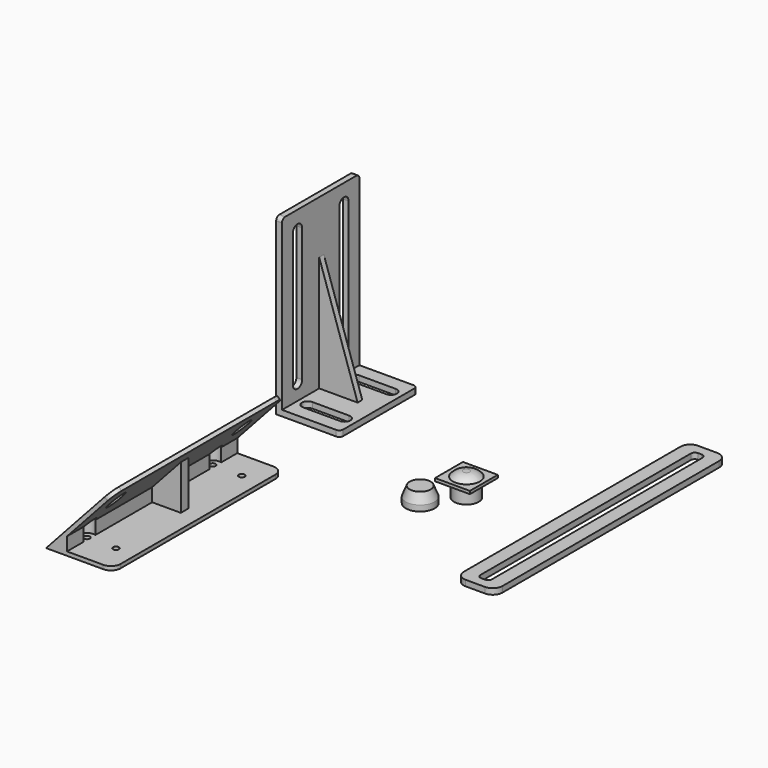
from build123d import *

# Parameters (mm, degrees)
F0_R        = 7
F1_DEPTH    = 2.5
F4_W        = 18
F4_H        = 18
F5_DEPTH    = 1.5
F7_R        = 6.4
F8_DEPTH    = 8
F9_R        = 7.45
F10_DEPTH   = 8
F11_SIZE2   = 5
F11_SIZE    = 2
F12_R       = 6.45
F13_DEPTH   = 7
F14_SIZE2   = 4
F14_SIZE    = 1.7
F17_DEPTH   = 3
F19_DEPTH   = 3
F20_W       = 3
F20_H       = 50
F21_DEPTH   = 90
F22_R       = 2
F24_DEPTH   = 25
F26_DEPTH   = 25
F29_DEPTH   = 3
F31_DEPTH   = 2
F33_DEPTH   = 110
F34_R       = 5
F36_DEPTH   = 110
F39_D       = 3
F39_DEPTH   = 50
F39_START   = 24.7920605
F39_START_2 = 41.2055101
F39_TIP     = 0.9012909285
F41_D       = 8
F41_DEPTH   = 19
F41_START   = 27.5276354
F41_START_2 = 43.9410851
F41_TIP     = 2.4034424761
F42_R       = 4
F43_DEPTH   = 2
F45_D       = 3
F45_DEPTH   = 19
F45_TIP     = 0.9012909285
F48_DEPTH   = 5


# Not quite as in the source:
# - a fillet or chamfer that OpenCascade refuses, or shapes differently, is made with other operations: its cross-section is extruded or revolved along the edge and cut away or added


with BuildPart() as f1:
    # F0 (on Top) → F1 (new body)
    with BuildSketch(Plane.XY):
        Circle(F0_R)
    extrude(amount=F1_DEPTH)

    # F2: fillet of radius 7 on 1 edges, made by hand

    # F2_s1 → F2_t2 (revolve, cut)
    with BuildSketch(Plane.XZ):
        with BuildLine():
            ThreePointArc((7, 0), (4.5961372442, 1.8442887702), (1.6380973526, 2.5))
            Line((1.6380973526, 2.5), (7, 2.5))
            Line((7, 2.5), (7, 0))
        make_face()
    revolve(axis=Axis((0, 0, 2.5), (0, 0, 1)), mode=Mode.SUBTRACT)

    # F4 (on offset) → F5 (join)
    with BuildSketch(Plane(origin=(0, 0, 0), x_dir=(1, 0, 0), z_dir=(0, 0, -1))):
        Rectangle(F4_W, F4_H)
    extrude(amount=F5_DEPTH)

    # F7 (on offset) → F8 (join)
    with BuildSketch(Plane(origin=(0, 0, -1.5), x_dir=(1, 0, 0), z_dir=(0, 0, -1))):
        Circle(F7_R)
    extrude(amount=F8_DEPTH)


with BuildPart() as f10:
    # F9 (on Top) → F10 (new body)
    with BuildSketch(Plane.XY):
        with Locations((0, -29.8365864904)):
            Circle(F9_R)
    extrude(amount=F10_DEPTH)

    # F11
    f11_edges = [f10.edges().sort_by_distance(p)[0] for p in [
        (-7.45, -29.836586, 8),
    ]]
    f11_side = f10.faces().sort_by_distance((0, -29.836586, 8))[0]
    chamfer(f11_edges, length=F11_SIZE, length2=F11_SIZE2, reference=f11_side)


with BuildPart() as f13:
    # F12 (on Top) → F13 (new body)
    with BuildSketch(Plane.XY):
        with Locations((0, -29.8365864904)):
            Circle(F12_R)
    extrude(amount=F13_DEPTH)

    # F14
    f14_edges = [f13.edges().sort_by_distance(p)[0] for p in [
        (-6.45, -29.836586, 7),
    ]]
    f14_side = f13.faces().sort_by_distance((0, -29.836586, 7))[0]
    chamfer(f14_edges, length=F14_SIZE, length2=F14_SIZE2, reference=f14_side)


with BuildPart() as f10_1:
    add(f10.part)

    # F15: cut F13
    add(f13.part, mode=Mode.SUBTRACT)


with BuildPart() as f17:
    # F16 (on Top) → F17 (new body)
    with BuildSketch(Plane.XY):
        with BuildLine():
            Line((69.802095294, 74.7819127334), (59.802095294, 74.7819127334))
            ThreePointArc((59.802095294, 74.7819127334), (56.2665613881, 73.3174466393), (54.802095294, 69.7819127334))
            Line((54.802095294, 69.7819127334), (54.802095294, -70.2180872666))
            ThreePointArc((54.802095294, -70.2180872666), (56.2665613881, -73.7536211725), (59.802095294, -75.2180872666))
            Line((59.802095294, -75.2180872666), (69.802095294, -75.2180872666))
            ThreePointArc((69.802095294, -75.2180872666), (73.3376291999, -73.7536211725), (74.802095294, -70.2180872666))
            Line((74.802095294, -70.2180872666), (74.802095294, 69.7819127334))
            ThreePointArc((74.802095294, 69.7819127334), (73.3376291999, 73.3174466393), (69.802095294, 74.7819127334))
        make_face()
        with BuildLine():
            ThreePointArc((61.802095294, 67.7819127334), (62.3878817316, 69.1961262958), (63.802095294, 69.7819127334))
            Line((63.802095294, 69.7819127334), (65.802095294, 69.7819127334))
            ThreePointArc((65.802095294, 69.7819127334), (67.2163088564, 69.1961262958), (67.802095294, 67.7819127334))
            Line((67.802095294, 67.7819127334), (67.802095294, -68.2180872666))
            ThreePointArc((67.802095294, -68.2180872666), (67.2163088564, -69.632300829), (65.802095294, -70.2180872666))
            Line((65.802095294, -70.2180872666), (63.802095294, -70.2180872666))
            ThreePointArc((63.802095294, -70.2180872666), (62.3878817316, -69.632300829), (61.802095294, -68.2180872666))
            Line((61.802095294, -68.2180872666), (61.802095294, 67.7819127334))
        make_face(mode=Mode.SUBTRACT)
    extrude(amount=F17_DEPTH)


with BuildPart() as f19:
    # F18 (on Top) → F19 (new body)
    with BuildSketch(Plane.XY):
        with BuildLine():
            Line((-62.8178298175, 44.4356946539), (-90.8178298175, 44.4356946539))
            Line((-90.8178298175, 44.4356946539), (-90.8178298175, -5.5643053461))
            Line((-90.8178298175, -5.5643053461), (-62.8178298175, -5.5643053461))
            ThreePointArc((-62.8178298175, -5.5643053461), (-61.4036162552, -4.9785189084), (-60.8178298175, -3.5643053461))
            Line((-60.8178298175, -3.5643053461), (-60.8178298175, 42.4356946539))
            ThreePointArc((-60.8178298175, 42.4356946539), (-61.4036162552, 43.8499082163), (-62.8178298175, 44.4356946539))
        make_face()
    extrude(amount=F19_DEPTH)

    # F20 (on Top) → F21 (join)
    with BuildSketch(Plane.XY):
        with Locations((-92.3178298175, 19.4356946539)):
            Rectangle(F20_W, F20_H)
    extrude(amount=F21_DEPTH)

    # F22
    f22_edges = [f19.edges().sort_by_distance(p)[0] for p in [
        (-92.31783, -5.564305, 90),
        (-92.31783, 44.435695, 90),
    ]]
    fillet(f22_edges, radius=F22_R)

    # F23 (on face) → F24 (cut)
    with BuildSketch(Plane.XY.offset(3)):
        with BuildLine():
            Line((-66.4884431298, 37.4356946539), (-85.4884431298, 37.4356946539))
            ThreePointArc((-85.4884431298, 37.4356946539), (-87.6097634734, 36.5570149975), (-88.4884431298, 34.4356946539))
            ThreePointArc((-88.4884431298, 34.4356946539), (-87.6097634734, 32.3143743104), (-85.4884431298, 31.4356946539))
            Line((-85.4884431298, 31.4356946539), (-66.4884431298, 31.4356946539))
            ThreePointArc((-66.4884431298, 31.4356946539), (-64.3671227862, 32.3143743104), (-63.4884431298, 34.4356946539))
            ThreePointArc((-63.4884431298, 34.4356946539), (-64.3671227862, 36.5570149975), (-66.4884431298, 37.4356946539))
        make_face()
        with BuildLine():
            Line((-66.4888298175, 7.4356946539), (-85.4888298175, 7.4356946539))
            ThreePointArc((-85.4888298175, 7.4356946539), (-87.6101501611, 6.5570149975), (-88.4888298175, 4.4356946539))
            ThreePointArc((-88.4888298175, 4.4356946539), (-87.6101501611, 2.3143743104), (-85.4888298175, 1.4356946539))
            Line((-85.4888298175, 1.4356946539), (-66.4888298175, 1.4356946539))
            ThreePointArc((-66.4888298175, 1.4356946539), (-64.367509474, 2.3143743104), (-63.4888298175, 4.4356946539))
            ThreePointArc((-63.4888298175, 4.4356946539), (-64.367509474, 6.5570149975), (-66.4888298175, 7.4356946539))
        make_face()
    extrude(amount=-F24_DEPTH, mode=Mode.SUBTRACT)

    # F25 (on face) → F26 (cut)
    with BuildSketch(Plane.YZ.offset(-90.8178298175)):
        with BuildLine():
            ThreePointArc((34.4356946539, 83.5), (32.3143743104, 82.6213203436), (31.4356946539, 80.5))
            Line((31.4356946539, 80.5), (31.4356946539, 11.5))
            ThreePointArc((31.4356946539, 11.5), (32.3143743104, 9.3786796564), (34.4356946539, 8.5))
            ThreePointArc((34.4356946539, 8.5), (36.5570149975, 9.3786796564), (37.4356946539, 11.5))
            Line((37.4356946539, 11.5), (37.4356946539, 80.5))
            ThreePointArc((37.4356946539, 80.5), (36.5570149975, 82.6213203436), (34.4356946539, 83.5))
        make_face()
        with BuildLine():
            ThreePointArc((4.4356946539, 83.5), (2.3143743104, 82.6213203436), (1.4356946539, 80.5))
            Line((1.4356946539, 80.5), (1.4356946539, 11.5))
            ThreePointArc((1.4356946539, 11.5), (2.3143743104, 9.3786796564), (4.4356946539, 8.5))
            ThreePointArc((4.4356946539, 8.5), (6.5570149975, 9.3786796564), (7.4356946539, 11.5))
            Line((7.4356946539, 11.5), (7.4356946539, 80.5))
            ThreePointArc((7.4356946539, 80.5), (6.5570149975, 82.6213203436), (4.4356946539, 83.5))
        make_face()
    extrude(amount=-F26_DEPTH, mode=Mode.SUBTRACT)

    # F28 (on face) → F29 (join)
    with BuildSketch(Plane.XZ.offset(-18.4356946539)):
        Polygon((-70.9541812539, 3), (-90.8178298175, 62.644213438), (-90.8178298175, 3), align=None)
    extrude(amount=-F29_DEPTH)


with BuildPart() as f31:
    # F30 (on Top) → F31 (new body)
    with BuildSketch(Plane.XY):
        with BuildLine():
            Line((-63.7690989673, -44.8433111385), (-88.7690989673, -44.8433111385))
            Line((-88.7690989673, -44.8433111385), (-88.7690989673, -154.8433111385))
            Line((-88.7690989673, -154.8433111385), (-63.7690989673, -154.8433111385))
            ThreePointArc((-63.7690989673, -154.8433111385), (-60.2335650614, -153.3788450445), (-58.7690989673, -149.8433111385))
            Line((-58.7690989673, -149.8433111385), (-58.7690989673, -49.8433111385))
            ThreePointArc((-58.7690989673, -49.8433111385), (-60.2335650614, -46.3077772326), (-63.7690989673, -44.8433111385))
        make_face()
    extrude(amount=F31_DEPTH)

    # F32 (on face) → F33 (join)
    with BuildSketch(Plane.XZ.offset(154.8433111385)):
        Polygon((-88.7690989673, 0), (-88.7690989673, 2), (-58.195712996, 35.4543153755), (-59.6720654413, 36.803531243), (-93.3062484509, 0), align=None)
    extrude(amount=-F33_DEPTH)

    # F34
    f34_edges = [f31.edges().sort_by_distance(p)[0] for p in [
        (-58.933889, -154.843311, 36.128923),
        (-58.933889, -44.843311, 36.128923),
    ]]
    fillet(f34_edges, radius=F34_R)

    # F35 (on face) → F36 (join)
    with BuildSketch(Plane.XZ.offset(154.8433111385)):
        Polygon((-82.4983428217, 8.8616493422), (-88.7690989673, 2), (-82.4983428217, 2), align=None)
    extrude(amount=-F36_DEPTH)

    # F39
    # its depths count from where the whole tool has entered the part; down to there all is cleared
    with Locations(Plane.XY.offset(50)):
        with Locations((-83.7690989673, -140.3433111385, -F39_START_2), (-68.7690989673, -140.3433111385, -F39_START), (-83.7690989673, -59.0733111385, -F39_START_2), (-68.7690989673, -59.0733111385, -F39_START)):
            Hole(F39_D / 2, depth=F39_DEPTH)
            with Locations((0, 0, -(F39_DEPTH + F39_TIP / 2))):  # 118° drill point
                Cone(0, F39_D / 2, F39_TIP, mode=Mode.SUBTRACT)

    # F41
    # its depths count from where the whole tool has entered the part; down to there all is cleared
    with Locations(Plane.XY.offset(50)):
        with Locations((-68.7690989673, -140.3433111385), (-68.7690989673, -59.0733111385)):
            Hole(F41_D / 2, depth=F41_START)
    with Locations(Plane.XY.offset(50)):
        with Locations((-83.7690989673, -140.3433111385), (-83.7690989673, -59.0733111385)):
            Hole(F41_D / 2, depth=F41_START_2)
    with Locations(Plane.XY.offset(50)):
        with Locations((-83.7690989673, -140.3433111385, -F41_START_2), (-68.7690989673, -140.3433111385, -F41_START), (-68.7690989673, -59.0733111385, -F41_START), (-83.7690989673, -59.0733111385, -F41_START_2)):
            Hole(F41_D / 2, depth=F41_DEPTH)
            with Locations((0, 0, -(F41_DEPTH + F41_TIP / 2))):  # 118° drill point
                Cone(0, F41_D / 2, F41_TIP, mode=Mode.SUBTRACT)

    # F42 (on face) → F43 (join)
    with BuildSketch(Plane(origin=(0, 0, 0), x_dir=(1, 0, 0), z_dir=(0, 0, -1))):
        with Locations((-83.7690989673, 59.0733111385)):
            Circle(F42_R)
        with Locations((-83.7690989673, 140.3433111385)):
            Circle(F42_R)
    extrude(amount=-F43_DEPTH)

    # F45
    with Locations(Plane.XY.offset(2)):
        with Locations((-83.7690989673, -59.0733111385), (-83.7690989673, -140.3433111385)):
            Hole(F45_D / 2, depth=F45_DEPTH)
            with Locations((0, 0, -(F45_DEPTH + F45_TIP / 2))):  # 118° drill point
                Cone(0, F45_D / 2, F45_TIP, mode=Mode.SUBTRACT)

    # F47 (on offset) → F48 (join)
    with BuildSketch(Plane.XZ.offset(99.8433111385)):
        Polygon((-82.4983428217, 2), (-67.6740757078, 2), (-67.6740757078, 25.0828067796), (-82.4983428217, 8.8616493422), align=None)
    extrude(amount=-F48_DEPTH)


solid = Compound([f1.part, f10_1.part, f17.part, f19.part, f31.part])
